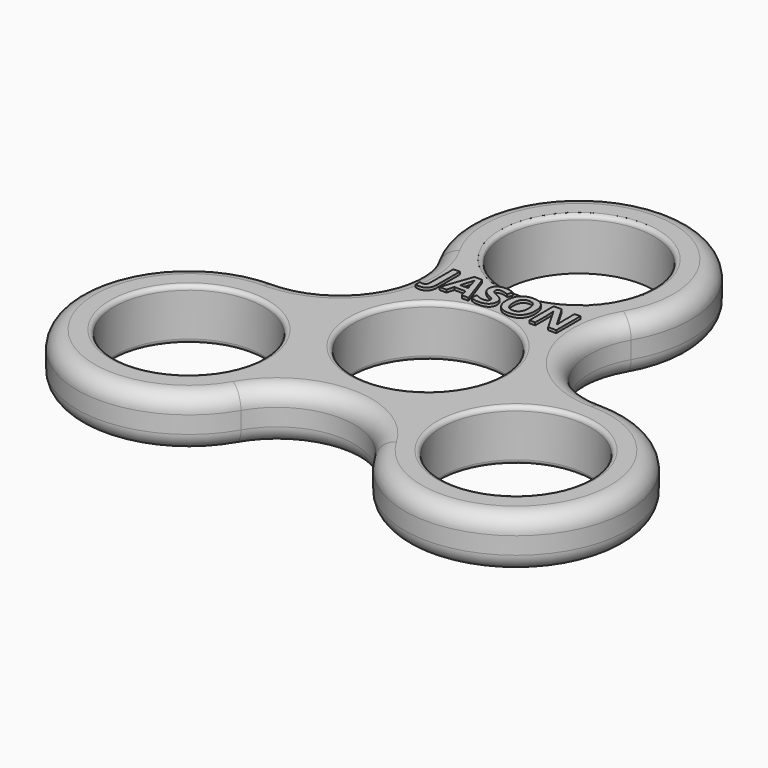
from build123d import *

# Parameters (mm, degrees)
F0_R         = 11.049
F1_DEPTH     = 7.62
F2_R         = 0.635
F3_R         = 2.54
F4_TEXT_SIZE = 6.2613771362
F5_DEPTH     = 0.396875


# Not quite as in the source:
# - Text() gives the source's letters only with a copy of the font that has no kerning and outlines rounded to 1/6400 em; it was checked with that copy


with BuildPart() as f1:
    # F0 (on Top) → F1 (new body)
    with BuildSketch(Plane.XY):
        with BuildLine():
            ThreePointArc((24.1967497817, 2.54), (14.2980794165, 8.255), (14.2980794165, 19.685))
            ThreePointArc((14.2980794165, 19.685), (0, 44.45), (-14.2980794165, 19.685))
            ThreePointArc((-14.2980794165, 19.685), (-14.2980794165, 8.255), (-24.1967497817, 2.54))
            ThreePointArc((-24.1967497817, 2.54), (-38.4948291982, -22.225), (-9.8986703653, -22.225))
            ThreePointArc((-9.8986703653, -22.225), (0, -16.51), (9.8986703653, -22.225))
            ThreePointArc((9.8986703653, -22.225), (38.4948291982, -22.225), (24.1967497817, 2.54))
        make_face()
        with Locations((-24.1967497817, -13.97)):
            Circle(F0_R, mode=Mode.SUBTRACT)
        with Locations((24.1967497817, -13.97)):
            Circle(F0_R, mode=Mode.SUBTRACT)
        Circle(F0_R, mode=Mode.SUBTRACT)
        with Locations((0, 27.94)):
            Circle(F0_R, mode=Mode.SUBTRACT)
    extrude(amount=F1_DEPTH)

    # F2
    f2_edges = [f1.edges().sort_by_distance(p)[0] for p in [
        (-11.049, 0, 7.62),
        (-11.049, 0, 0),
        (13.14775, -13.97, 0),
        (-35.24575, -13.97, 0),
        (-35.24575, -13.97, 7.62),
        (13.14775, -13.97, 7.62),
        (-11.049, 27.94, 7.62),
    ]]
    fillet(f2_edges, radius=F2_R)

    # F3
    f3_edges = [f1.edges().sort_by_distance(p)[0] for p in [
        (-38.494829, -22.225, 7.62),
        (-38.494829, -22.225, 0),
    ]]
    fillet(f3_edges, radius=F3_R)

    # F4 (on face) → F5 (join)
    with BuildSketch(Plane.XY.offset(7.62)):
        with Locations((-9.8305548362, 11.8167391834)):
            Text('JASON', F4_TEXT_SIZE, font='Open Sans', font_style=FontStyle.BOLD, text_align=(TextAlign.LEFT, TextAlign.BOTTOM))
    extrude(amount=F5_DEPTH)


solid = f1.part
